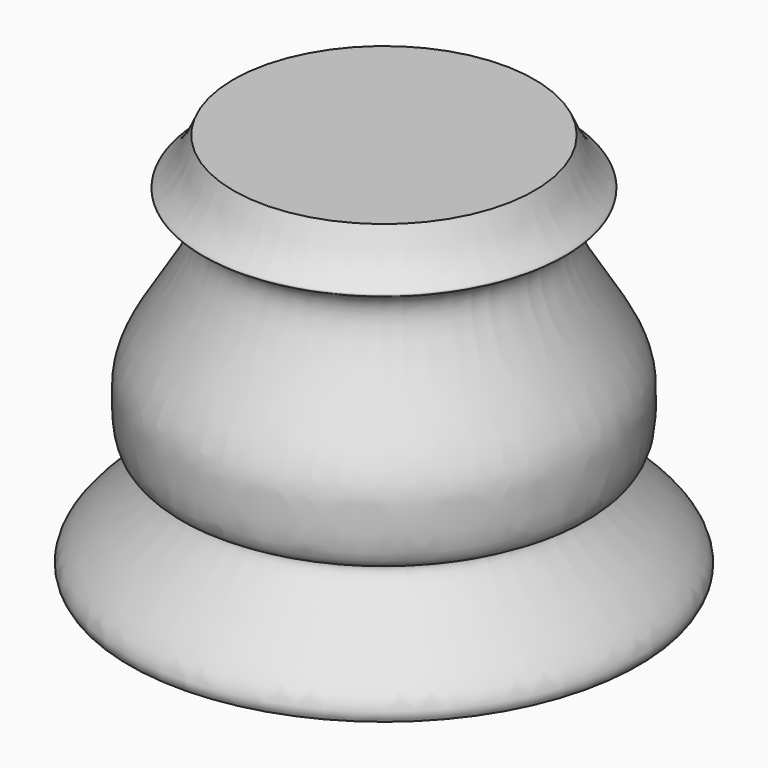
from build123d import *


with BuildPart() as f2:
    # F0 (on Front) → F2 (revolve)
    with BuildSketch(Plane.XZ):
        with BuildLine():
            Line((0, 27.7682077042), (-5.3002026468, 27.7682077042))
            add(Edge.make_bspline(
                [(-5.3002026468, 27.7682077042), (-5.4605062478, 27.3616354465), (-5.9627121178, 26.3310907989), (-6.7918361778, 26.1262496351), (-5.2170696756, 25.6909190192), (-5.2183445861, 24.0749700794), (-7.4856064998, 21.1514288504), (-7.4873686315, 19.7136508406), (-7.4592975783, 17.9435108088), (-5.9023238156, 17.8655136182), (-6.89405113, 16.5827279586), (-9.3976303075, 14.9604288728), (-8.9747941843, 14.2645384553), (-8.9591628024, 14.24242636)],
                knots=[0.253490364, 0.253490364, 0.253490364, 0.253490364, 0.2770069123, 0.3248848799, 0.3750325074, 0.4338287084, 0.529700376, 0.5922757431, 0.6536436214, 0.7027449596, 0.7585125505, 0.8480046848, 0.8509865829, 0.8509865829, 0.8509865829, 0.8509865829], degree=3))
            Line((-8.9591628024, 14.24242636), (0, 14.2019145489))
            Line((0, 14.2019145489), (0, 26.5156850219))
            Line((0, 26.5156850219), (0, 27.7682077042))
        make_face()
    revolve(axis=Axis((0, 0, 28.1776376069), (0, 0, -1)))


solid = f2.part
